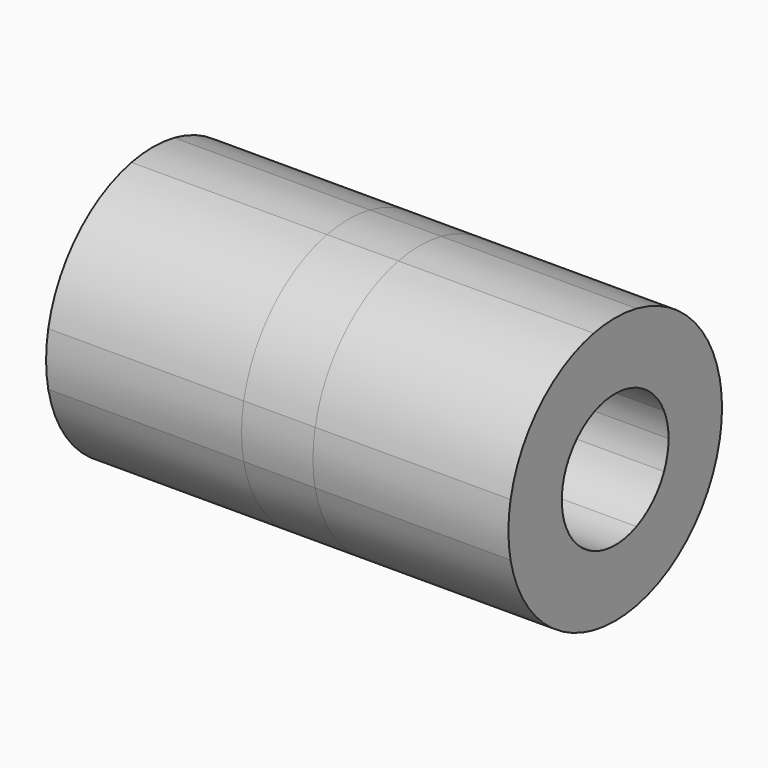
from build123d import *

# Parameters (mm, degrees)
F1_DEPTH = 25.4
F2_DEPTH = 44.00509


# Not quite as in the source:
# - a pattern or mirror of a feature is missing from the dataset's text; its kind, count and spacing are read off the source's solid
# - a feature names something its author has since deleted; it is built from what else it names


with BuildPart() as f1:
    # F0 (on Right) → F1 (new body)
    with BuildSketch(Plane.YZ):
        with BuildLine():
            ThreePointArc((12.4434078933, -2.54), (12.6356891432, -1.2764638175), (12.7, 0))
            ThreePointArc((12.7, 0), (12.6356891432, 1.2764638175), (12.4434078933, 2.54))
            Line((12.4434078933, 2.54), (5.8198711326, 2.54))
            ThreePointArc((5.8198711326, 2.54), (6.2160550871, 1.2973662374), (6.35, 0))
            ThreePointArc((6.35, 0), (6.2160550871, -1.2973662374), (5.8198711326, -2.54))
            Line((5.8198711326, -2.54), (12.4434078933, -2.54))
        make_face()
        with BuildLine():
            Line((5.8198711326, 2.54), (12.4434078933, 2.54))
            ThreePointArc((12.4434078933, 2.54), (8.9802561211, 8.9802561211), (2.54, 12.4434078933))
            Line((2.54, 12.4434078933), (2.54, 5.8198711326))
            ThreePointArc((2.54, 5.8198711326), (4.4901280605, 4.4901280605), (5.8198711326, 2.54))
        make_face()
        with BuildLine():
            ThreePointArc((2.54, -12.4434078933), (8.9802561211, -8.9802561211), (12.4434078933, -2.54))
            Line((12.4434078933, -2.54), (5.8198711326, -2.54))
            ThreePointArc((5.8198711326, -2.54), (4.4901280605, -4.4901280605), (2.54, -5.8198711326))
            Line((2.54, -5.8198711326), (2.54, -12.4434078933))
        make_face()
        with BuildLine():
            Line((2.54, 5.8198711326), (2.54, 12.4434078933))
            ThreePointArc((2.54, 12.4434078933), (0, 12.7), (-2.54, 12.4434078933))
            Line((-2.54, 12.4434078933), (-2.54, 5.8198711326))
            ThreePointArc((-2.54, 5.8198711326), (0, 6.35), (2.54, 5.8198711326))
        make_face()
        with BuildLine():
            ThreePointArc((-2.54, -12.4434078933), (0, -12.7), (2.54, -12.4434078933))
            Line((2.54, -12.4434078933), (2.54, -5.8198711326))
            ThreePointArc((2.54, -5.8198711326), (0, -6.35), (-2.54, -5.8198711326))
            Line((-2.54, -5.8198711326), (-2.54, -12.4434078933))
        make_face()
        with BuildLine():
            Line((-2.54, 5.8198711326), (-2.54, 12.4434078933))
            ThreePointArc((-2.54, 12.4434078933), (-8.9802561211, 8.9802561211), (-12.4434078933, 2.54))
            Line((-12.4434078933, 2.54), (-5.8198711326, 2.54))
            ThreePointArc((-5.8198711326, 2.54), (-4.4901280605, 4.4901280605), (-2.54, 5.8198711326))
        make_face()
        with BuildLine():
            ThreePointArc((-12.4434078933, -2.54), (-8.9802561211, -8.9802561211), (-2.54, -12.4434078933))
            Line((-2.54, -12.4434078933), (-2.54, -5.8198711326))
            ThreePointArc((-2.54, -5.8198711326), (-4.4901280605, -4.4901280605), (-5.8198711326, -2.54))
            Line((-5.8198711326, -2.54), (-12.4434078933, -2.54))
        make_face()
        with BuildLine():
            Line((-5.8198711326, 2.54), (-12.4434078933, 2.54))
            ThreePointArc((-12.4434078933, 2.54), (-12.7, 0), (-12.4434078933, -2.54))
            Line((-12.4434078933, -2.54), (-5.8198711326, -2.54))
            ThreePointArc((-5.8198711326, -2.54), (-6.35, 0), (-5.8198711326, 2.54))
        make_face()
    extrude(amount=F1_DEPTH)

    # F1_copies: F1 across plane


with BuildPart() as f1_1:
    add(f1.part)
    add(f1.part.mirror(Plane(origin=(22.002045, 0, 0), x_dir=(0, 0, 1), z_dir=(1, 0, 0))))

    # F0 (on Right) → F2 (join, through all)
    with BuildSketch(Plane.YZ):
        with BuildLine():
            ThreePointArc((12.4434078933, -2.54), (12.6356891432, -1.2764638175), (12.7, 0))
            ThreePointArc((12.7, 0), (12.6356891432, 1.2764638175), (12.4434078933, 2.54))
            Line((12.4434078933, 2.54), (5.8198711326, 2.54))
            ThreePointArc((5.8198711326, 2.54), (6.2160550871, 1.2973662374), (6.35, 0))
            ThreePointArc((6.35, 0), (6.2160550871, -1.2973662374), (5.8198711326, -2.54))
            Line((5.8198711326, -2.54), (12.4434078933, -2.54))
        make_face()
        with BuildLine():
            Line((5.8198711326, 2.54), (12.4434078933, 2.54))
            ThreePointArc((12.4434078933, 2.54), (8.9802561211, 8.9802561211), (2.54, 12.4434078933))
            Line((2.54, 12.4434078933), (2.54, 5.8198711326))
            ThreePointArc((2.54, 5.8198711326), (4.4901280605, 4.4901280605), (5.8198711326, 2.54))
        make_face()
        with BuildLine():
            ThreePointArc((2.54, -12.4434078933), (8.9802561211, -8.9802561211), (12.4434078933, -2.54))
            Line((12.4434078933, -2.54), (5.8198711326, -2.54))
            ThreePointArc((5.8198711326, -2.54), (4.4901280605, -4.4901280605), (2.54, -5.8198711326))
            Line((2.54, -5.8198711326), (2.54, -12.4434078933))
        make_face()
        with BuildLine():
            Line((2.54, 5.8198711326), (2.54, 12.4434078933))
            ThreePointArc((2.54, 12.4434078933), (0, 12.7), (-2.54, 12.4434078933))
            Line((-2.54, 12.4434078933), (-2.54, 5.8198711326))
            ThreePointArc((-2.54, 5.8198711326), (0, 6.35), (2.54, 5.8198711326))
        make_face()
        with BuildLine():
            ThreePointArc((-2.54, -12.4434078933), (0, -12.7), (2.54, -12.4434078933))
            Line((2.54, -12.4434078933), (2.54, -5.8198711326))
            ThreePointArc((2.54, -5.8198711326), (0, -6.35), (-2.54, -5.8198711326))
            Line((-2.54, -5.8198711326), (-2.54, -12.4434078933))
        make_face()
        with BuildLine():
            Line((-2.54, 5.8198711326), (-2.54, 12.4434078933))
            ThreePointArc((-2.54, 12.4434078933), (-8.9802561211, 8.9802561211), (-12.4434078933, 2.54))
            Line((-12.4434078933, 2.54), (-5.8198711326, 2.54))
            ThreePointArc((-5.8198711326, 2.54), (-4.4901280605, 4.4901280605), (-2.54, 5.8198711326))
        make_face()
        with BuildLine():
            ThreePointArc((-12.4434078933, -2.54), (-8.9802561211, -8.9802561211), (-2.54, -12.4434078933))
            Line((-2.54, -12.4434078933), (-2.54, -5.8198711326))
            ThreePointArc((-2.54, -5.8198711326), (-4.4901280605, -4.4901280605), (-5.8198711326, -2.54))
            Line((-5.8198711326, -2.54), (-12.4434078933, -2.54))
        make_face()
        with BuildLine():
            Line((-5.8198711326, 2.54), (-12.4434078933, 2.54))
            ThreePointArc((-12.4434078933, 2.54), (-12.7, 0), (-12.4434078933, -2.54))
            Line((-12.4434078933, -2.54), (-5.8198711326, -2.54))
            ThreePointArc((-5.8198711326, -2.54), (-6.35, 0), (-5.8198711326, 2.54))
        make_face()
    extrude(amount=F2_DEPTH)


solid = f1_1.part
